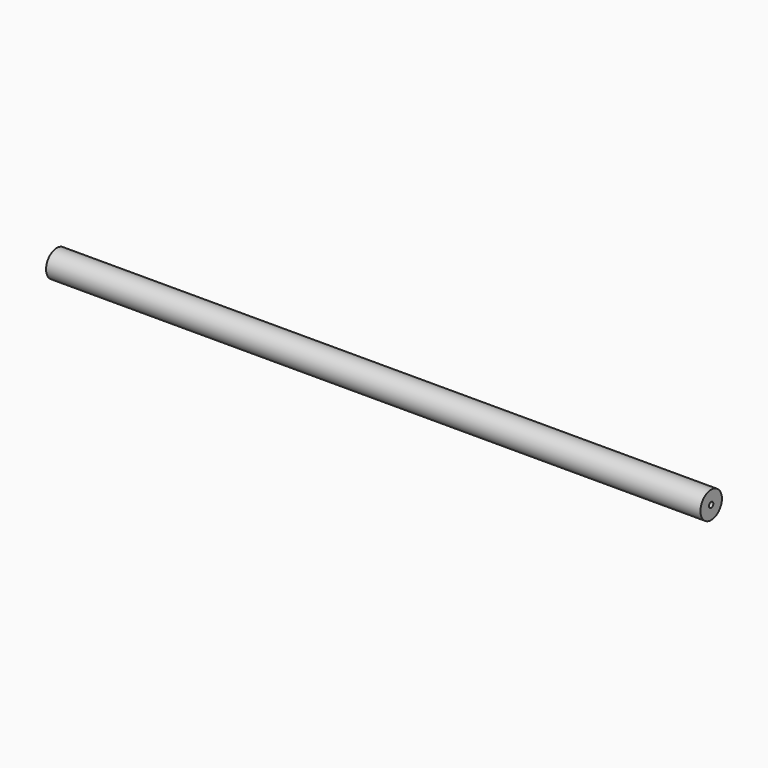
from build123d import *

# Parameters (mm, degrees)
F0_R           = 12.5
F1_DEPTH       = 304.5
F4_D           = 5
F4_DEPTH       = 18
F4_TIP         = 1.5021515476
F4_ON_F2_D     = 5
F4_ON_F2_DEPTH = 18
F4_ON_F2_TIP   = 1.5021515476


with BuildPart() as f1:
    # F0 (on Right) → F1 (new body, symmetric)
    with BuildSketch(Plane.YZ):
        Circle(F0_R)
    extrude(amount=F1_DEPTH, both=True)

    # F4
    with Locations(Plane(origin=(-304.5, 0, 0), x_dir=(0, -1, 0), z_dir=(-1, 0, 0))):
        with Locations((0, 0)):
            Hole(F4_D / 2, depth=F4_DEPTH)
            with Locations((0, 0, -(F4_DEPTH + F4_TIP / 2))):  # 118° drill point
                Cone(0, F4_D / 2, F4_TIP, mode=Mode.SUBTRACT)

    # F4 on F2
    with Locations(Plane.YZ.offset(304.5)):
        with Locations((0, 0)):
            Hole(F4_ON_F2_D / 2, depth=F4_ON_F2_DEPTH)
            with Locations((0, 0, -(F4_ON_F2_DEPTH + F4_ON_F2_TIP / 2))):  # 118° drill point
                Cone(0, F4_ON_F2_D / 2, F4_ON_F2_TIP, mode=Mode.SUBTRACT)


solid = f1.part
